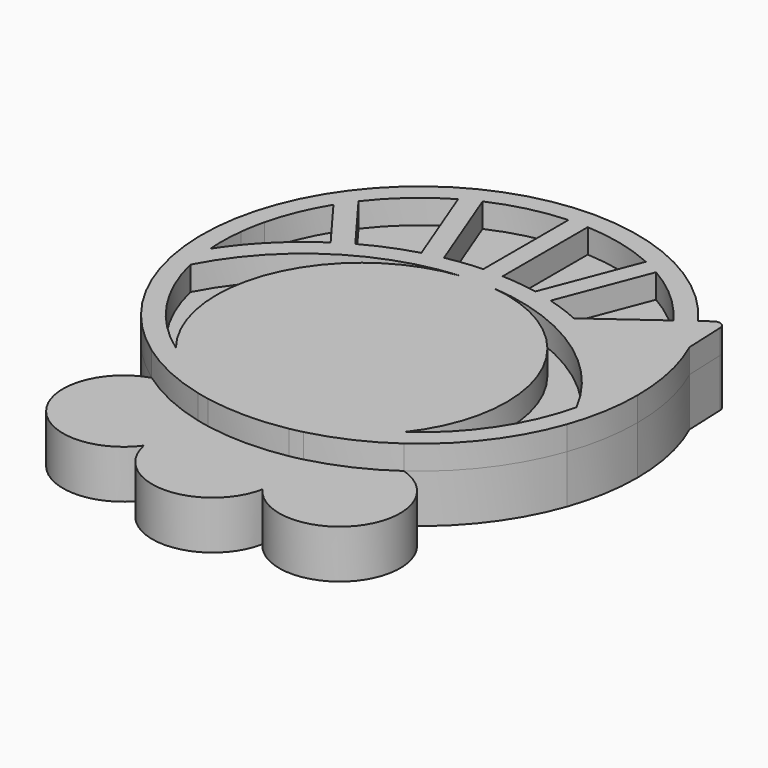
from build123d import *

# Parameters (mm, degrees)
F1_DEPTH = 2
F2_DEPTH = 1


with BuildPart() as f1:
    # F0 (on Top) → F1 (new body)
    with BuildSketch(Plane.XY):
        with BuildLine():
            ThreePointArc((7.2814781438, 5.28961965), (-6.3961147037, 6.3316440753), (-5.2155835522, -7.3346907372))
            ThreePointArc((-5.2155835522, -7.3346907372), (-3.7605276418, -8.1767005482), (-2.1742632903, -8.7334173806))
            ThreePointArc((-2.1742632903, -8.7334173806), (-1.9247980499, -8.7917661745), (-1.6737730699, -8.8429906542))
            ThreePointArc((-1.6737730699, -8.8429906542), (0, -9), (1.6737730699, -8.8429906542))
            ThreePointArc((1.6737730699, -8.8429906542), (1.9247980499, -8.7917661745), (2.1742632903, -8.7334173806))
            ThreePointArc((2.1742632903, -8.7334173806), (3.7605276418, -8.1767005482), (5.2155835522, -7.3346907372))
            ThreePointArc((5.2155835522, -7.3346907372), (7.1851103596, -5.4197960404), (8.4852813742, -3))
            Line((8.4852813742, -3), (8.2074613141, 3.6929092566))
            ThreePointArc((8.2074613141, 3.6929092566), (7.785511056, 4.5150656249), (7.2814781438, 5.28961965))
        make_face()
        with BuildLine():
            ThreePointArc((4.0924321005, 7.1057722664), (5.4838115432, 6.0965409011), (6.6342356421, 4.8194312366))
            ThreePointArc((6.6342356421, 4.8194312366), (7.7987413172, 2.5336996403), (8.2, 0))
            ThreePointArc((8.2, 0), (8.1945029875, -0.3002012451), (8.1780193201, -0.6))
            ThreePointArc((8.1780193201, -0.6), (8.1056933876, -1.2400543156), (7.9833517385, -1.8724569471))
            ThreePointArc((7.9833517385, -1.8724569471), (6.7951614423, -4.5897473758), (4.718116385, -6.7066666667))
            ThreePointArc((4.718116385, -6.7066666667), (0, -8.2), (-4.718116385, -6.7066666667))
            ThreePointArc((-4.718116385, -6.7066666667), (-6.7951614423, -4.5897473758), (-7.9833517385, -1.8724569471))
            ThreePointArc((-7.9833517385, -1.8724569471), (-8.1056933876, -1.2400543156), (-8.1780193201, -0.6))
            ThreePointArc((-8.1780193201, -0.6), (-8.19816566, 0.1734353216), (-8.1453273459, 0.945326625))
            ThreePointArc((-8.1453273459, 0.945326625), (-8.071860174, 1.4439783003), (-7.9678953297, 1.9371742346))
            ThreePointArc((-7.9678953297, 1.9371742346), (-7.5714581737, 3.148495057), (-6.992101102, 4.2837509475))
            ThreePointArc((-6.992101102, 4.2837509475), (-6.7619721437, 4.6385054412), (-6.5138611979, 4.9809248433))
            ThreePointArc((-6.5138611979, 4.9809248433), (-5.408521843, 6.1634317936), (-4.0924321005, 7.1057722664))
            ThreePointArc((-4.0924321005, 7.1057722664), (-3.7389698581, 7.2979520689), (-3.3765066945, 7.4725633181))
            ThreePointArc((-3.3765066945, 7.4725633181), (-1.9220470789, 7.9715578795), (-0.4, 8.1902380918))
            ThreePointArc((-0.4, 8.1902380918), (0, 8.2), (0.4, 8.1902380918))
            ThreePointArc((0.4, 8.1902380918), (1.9220470789, 7.9715578795), (3.3765066945, 7.4725633181))
            ThreePointArc((3.3765066945, 7.4725633181), (3.7389698581, 7.2979520689), (4.0924321005, 7.1057722664))
        make_face(mode=Mode.SUBTRACT)
        with BuildLine():
            ThreePointArc((-4.718116385, -6.7066666667), (0, -8.2), (4.718116385, -6.7066666667))
            ThreePointArc((4.718116385, -6.7066666667), (5.5357708849, -0.6858606979), (0.6763903311, 2.9617527725))
            ThreePointArc((0.6763903311, 2.9617527725), (0, 2.9872418814), (-0.6763903311, 2.9617527725))
            ThreePointArc((-0.6763903311, 2.9617527725), (-5.5357708849, -0.6858606979), (-4.718116385, -6.7066666667))
        make_face()
        with BuildLine():
            ThreePointArc((-2.1742632903, -8.7334173806), (-3.7605276418, -8.1767005482), (-5.2155835522, -7.3346907372))
            ThreePointArc((-5.2155835522, -7.3346907372), (-6.5031269408, -11.1771583895), (-2.4507149007, -11.1939599938))
            ThreePointArc((-2.4507149007, -11.1939599938), (-2.4421572707, -10.165333875), (-2.020134629, -9.2272284357))
            ThreePointArc((-2.020134629, -9.2272284357), (-2.0843920362, -8.976325602), (-2.1742632903, -8.7334173806))
        make_face()
        with BuildLine():
            ThreePointArc((2.020134629, -9.2272284357), (2.4421572707, -10.165333875), (2.4507149007, -11.1939599938))
            ThreePointArc((2.4507149007, -11.1939599938), (6.5031269408, -11.1771583895), (5.2155835522, -7.3346907372))
            ThreePointArc((5.2155835522, -7.3346907372), (3.7605276418, -8.1767005482), (2.1742632903, -8.7334173806))
            ThreePointArc((2.1742632903, -8.7334173806), (2.0843920362, -8.976325602), (2.020134629, -9.2272284357))
        make_face()
        with BuildLine():
            ThreePointArc((-2.020134629, -9.2272284357), (-2.028692259, -10.2558545545), (-2.4507149007, -11.1939599938))
            ThreePointArc((-2.4507149007, -11.1939599938), (0, -13.2), (2.4507149007, -11.1939599938))
            ThreePointArc((2.4507149007, -11.1939599938), (2.028692259, -10.2558545545), (2.020134629, -9.2272284357))
            ThreePointArc((2.020134629, -9.2272284357), (1.8569190048, -9.0261267044), (1.6737730699, -8.8429906542))
            ThreePointArc((1.6737730699, -8.8429906542), (0, -9), (-1.6737730699, -8.8429906542))
            ThreePointArc((-1.6737730699, -8.8429906542), (-1.8569190048, -9.0261267044), (-2.020134629, -9.2272284357))
        make_face()
        with BuildLine():
            ThreePointArc((8.1780193201, -0.6), (6.3564187379, 1.4589503838), (4.0346237711, 2.9309468158))
            ThreePointArc((4.0346237711, 2.9309468158), (3.3625359736, 3.2050720707), (2.6720023112, 3.4287010584))
            ThreePointArc((2.6720023112, 3.4287010584), (2.2814259241, 3.5307447638), (1.8869783621, 3.6166164872))
            ThreePointArc((1.8869783621, 3.6166164872), (1.1468403301, 3.732664448), (0.4, 3.7918333319))
            ThreePointArc((0.4, 3.7918333319), (0, 3.8), (-0.4, 3.7918333319))
            ThreePointArc((-0.4, 3.7918333319), (-1.1468403301, 3.732664448), (-1.8869783621, 3.6166164872))
            ThreePointArc((-1.8869783621, 3.6166164872), (-2.2814259241, 3.5307447638), (-2.6720023112, 3.4287010584))
            ThreePointArc((-2.6720023112, 3.4287010584), (-3.7242179593, 3.0647780222), (-4.7283647591, 2.5838550026))
            ThreePointArc((-4.7283647591, 2.5838550026), (-5.0763601287, 2.382754192), (-5.4158169003, 2.1675533241))
            ThreePointArc((-5.4158169003, 2.1675533241), (-6.2373110314, 1.5588326544), (-6.9909121579, 0.8678342439))
            ThreePointArc((-6.9909121579, 0.8678342439), (-7.2666228528, 0.5754233563), (-7.530112508, 0.2719538915))
            ThreePointArc((-7.530112508, 0.2719538915), (-7.8661570846, -0.1550386896), (-8.1780193201, -0.6))
            ThreePointArc((-8.1780193201, -0.6), (-8.1056933876, -1.2400543156), (-7.9833517385, -1.8724569471))
            ThreePointArc((-7.9833517385, -1.8724569471), (-4.9588485641, 1.4953543981), (-0.6763903311, 2.9617527725))
            ThreePointArc((-0.6763903311, 2.9617527725), (0, 2.9872418814), (0.6763903311, 2.9617527725))
            ThreePointArc((0.6763903311, 2.9617527725), (4.9588485641, 1.4953543981), (7.9833517385, -1.8724569471))
            ThreePointArc((7.9833517385, -1.8724569471), (8.1056933876, -1.2400543156), (8.1780193201, -0.6))
        make_face()
        with BuildLine():
            ThreePointArc((4.718116385, -6.7066666667), (6.7951614423, -4.5897473758), (7.9833517385, -1.8724569471))
            ThreePointArc((7.9833517385, -1.8724569471), (4.9588485641, 1.4953543981), (0.6763903311, 2.9617527725))
            ThreePointArc((0.6763903311, 2.9617527725), (5.5357708849, -0.6858606979), (4.718116385, -6.7066666667))
        make_face()
        with BuildLine():
            ThreePointArc((-7.9833517385, -1.8724569471), (-6.7951614423, -4.5897473758), (-4.718116385, -6.7066666667))
            ThreePointArc((-4.718116385, -6.7066666667), (-5.5357708849, -0.6858606979), (-0.6763903311, 2.9617527725))
            ThreePointArc((-0.6763903311, 2.9617527725), (-4.9588485641, 1.4953543981), (-7.9833517385, -1.8724569471))
        make_face()
        with BuildLine():
            Line((1.8869783621, 3.6166164872), (3.3765066945, 7.4725633181))
            ThreePointArc((3.3765066945, 7.4725633181), (1.9220470789, 7.9715578795), (0.4, 8.1902380918))
            Line((0.4, 8.1902380918), (0.4, 3.7918333319))
            ThreePointArc((0.4, 3.7918333319), (1.1468403301, 3.732664448), (1.8869783621, 3.6166164872))
        make_face()
        with BuildLine():
            Line((-0.4, 3.7918333319), (-0.4, 8.1902380918))
            ThreePointArc((-0.4, 8.1902380918), (-1.9220470789, 7.9715578795), (-3.3765066945, 7.4725633181))
            Line((-3.3765066945, 7.4725633181), (-1.8869783621, 3.6166164872))
            ThreePointArc((-1.8869783621, 3.6166164872), (-1.1468403301, 3.732664448), (-0.4, 3.7918333319))
        make_face()
        with BuildLine():
            Line((-2.6720023112, 3.4287010584), (-4.0924321005, 7.1057722664))
            ThreePointArc((-4.0924321005, 7.1057722664), (-5.408521843, 6.1634317936), (-6.5138611979, 4.9809248433))
            Line((-6.5138611979, 4.9809248433), (-4.7283647591, 2.5838550026))
            ThreePointArc((-4.7283647591, 2.5838550026), (-3.7242179593, 3.0647780222), (-2.6720023112, 3.4287010584))
        make_face()
        with BuildLine():
            ThreePointArc((8.2, 0), (7.7987413172, 2.5336996403), (6.6342356421, 4.8194312366))
            Line((6.6342356421, 4.8194312366), (4.0346237711, 2.9309468158))
            ThreePointArc((4.0346237711, 2.9309468158), (6.3564187379, 1.4589503838), (8.1780193201, -0.6))
            ThreePointArc((8.1780193201, -0.6), (8.1945029875, -0.3002012451), (8.2, 0))
        make_face()
        with BuildLine():
            Line((4.0346237711, 2.9309468158), (6.6342356421, 4.8194312366))
            ThreePointArc((6.6342356421, 4.8194312366), (5.4838115432, 6.0965409011), (4.0924321005, 7.1057722664))
            Line((4.0924321005, 7.1057722664), (2.6720023112, 3.4287010584))
            ThreePointArc((2.6720023112, 3.4287010584), (3.3625359736, 3.2050720707), (4.0346237711, 2.9309468158))
        make_face()
        with BuildLine():
            Line((-5.4158169003, 2.1675533241), (-6.992101102, 4.2837509475))
            ThreePointArc((-6.992101102, 4.2837509475), (-7.5714581737, 3.148495057), (-7.9678953297, 1.9371742346))
            Line((-7.9678953297, 1.9371742346), (-6.9909121579, 0.8678342439))
            ThreePointArc((-6.9909121579, 0.8678342439), (-6.2373110314, 1.5588326544), (-5.4158169003, 2.1675533241))
        make_face()
        with BuildLine():
            Line((0.4, 3.7918333319), (0.4, 8.1902380918))
            ThreePointArc((0.4, 8.1902380918), (0, 8.2), (-0.4, 8.1902380918))
            Line((-0.4, 8.1902380918), (-0.4, 3.7918333319))
            ThreePointArc((-0.4, 3.7918333319), (0, 3.8), (0.4, 3.7918333319))
        make_face()
        with BuildLine():
            Line((2.6720023112, 3.4287010584), (4.0924321005, 7.1057722664))
            ThreePointArc((4.0924321005, 7.1057722664), (3.7389698581, 7.2979520689), (3.3765066945, 7.4725633181))
            Line((3.3765066945, 7.4725633181), (1.8869783621, 3.6166164872))
            ThreePointArc((1.8869783621, 3.6166164872), (2.2814259241, 3.5307447638), (2.6720023112, 3.4287010584))
        make_face()
        with BuildLine():
            Line((-1.8869783621, 3.6166164872), (-3.3765066945, 7.4725633181))
            ThreePointArc((-3.3765066945, 7.4725633181), (-3.7389698581, 7.2979520689), (-4.0924321005, 7.1057722664))
            Line((-4.0924321005, 7.1057722664), (-2.6720023112, 3.4287010584))
            ThreePointArc((-2.6720023112, 3.4287010584), (-2.2814259241, 3.5307447638), (-1.8869783621, 3.6166164872))
        make_face()
        with BuildLine():
            ThreePointArc((9, 0), (8.7996349875, 1.8884978387), (8.2074613141, 3.6929092566))
            Line((8.2074613141, 3.6929092566), (8.4852813742, -3))
            ThreePointArc((8.4852813742, -3), (8.8703870369, -1.5219178085), (9, 0))
        make_face()
        with BuildLine():
            Line((-4.7283647591, 2.5838550026), (-6.5138611979, 4.9809248433))
            ThreePointArc((-6.5138611979, 4.9809248433), (-6.7619721437, 4.6385054412), (-6.992101102, 4.2837509475))
            Line((-6.992101102, 4.2837509475), (-5.4158169003, 2.1675533241))
            ThreePointArc((-5.4158169003, 2.1675533241), (-5.0763601287, 2.382754192), (-4.7283647591, 2.5838550026))
        make_face()
        with BuildLine():
            ThreePointArc((-7.9678953297, 1.9371742346), (-8.071860174, 1.4439783003), (-8.1453273459, 0.945326625))
            Line((-8.1453273459, 0.945326625), (-7.530112508, 0.2719538915))
            ThreePointArc((-7.530112508, 0.2719538915), (-7.2666228528, 0.5754233563), (-6.9909121579, 0.8678342439))
            Line((-6.9909121579, 0.8678342439), (-7.9678953297, 1.9371742346))
        make_face()
        with BuildLine():
            Line((7.6860047074, 5.5834874083), (7.2814781438, 5.28961965))
            ThreePointArc((7.2814781438, 5.28961965), (7.785511056, 4.5150656249), (8.2074613141, 3.6929092566))
            Line((8.2074613141, 3.6929092566), (8.1380607123, 5.3648257129))
            ThreePointArc((8.1380607123, 5.3648257129), (7.9774785182, 5.6094576733), (7.6860047074, 5.5834874083))
        make_face()
        with BuildLine():
            ThreePointArc((-2.020134629, -9.2272284357), (-2.4421572707, -10.165333875), (-2.4507149007, -11.1939599938))
            ThreePointArc((-2.4507149007, -11.1939599938), (-2.028692259, -10.2558545545), (-2.020134629, -9.2272284357))
        make_face()
        with BuildLine():
            ThreePointArc((2.020134629, -9.2272284357), (2.028692259, -10.2558545545), (2.4507149007, -11.1939599938))
            ThreePointArc((2.4507149007, -11.1939599938), (2.4421572707, -10.165333875), (2.020134629, -9.2272284357))
        make_face()
        with BuildLine():
            ThreePointArc((-8.1453273459, 0.945326625), (-8.19816566, 0.1734353216), (-8.1780193201, -0.6))
            ThreePointArc((-8.1780193201, -0.6), (-7.8661570846, -0.1550386896), (-7.530112508, 0.2719538915))
            Line((-7.530112508, 0.2719538915), (-8.1453273459, 0.945326625))
        make_face()
        with BuildLine():
            ThreePointArc((-1.6737730699, -8.8429906542), (-1.9247980499, -8.7917661745), (-2.1742632903, -8.7334173806))
            ThreePointArc((-2.1742632903, -8.7334173806), (-2.0843920362, -8.976325602), (-2.020134629, -9.2272284357))
            ThreePointArc((-2.020134629, -9.2272284357), (-1.8569190048, -9.0261267044), (-1.6737730699, -8.8429906542))
        make_face()
        with BuildLine():
            ThreePointArc((2.1742632903, -8.7334173806), (1.9247980499, -8.7917661745), (1.6737730699, -8.8429906542))
            ThreePointArc((1.6737730699, -8.8429906542), (1.8569190048, -9.0261267044), (2.020134629, -9.2272284357))
            ThreePointArc((2.020134629, -9.2272284357), (2.0843920362, -8.976325602), (2.1742632903, -8.7334173806))
        make_face()
    extrude(amount=F1_DEPTH)


with BuildPart() as f2:
    # F0 (on Top) → F2 (new body)
    with BuildSketch(Plane.XY):
        with BuildLine():
            ThreePointArc((7.2814781438, 5.28961965), (-6.3961147037, 6.3316440753), (-5.2155835522, -7.3346907372))
            ThreePointArc((-5.2155835522, -7.3346907372), (-3.7605276418, -8.1767005482), (-2.1742632903, -8.7334173806))
            ThreePointArc((-2.1742632903, -8.7334173806), (-1.9247980499, -8.7917661745), (-1.6737730699, -8.8429906542))
            ThreePointArc((-1.6737730699, -8.8429906542), (0, -9), (1.6737730699, -8.8429906542))
            ThreePointArc((1.6737730699, -8.8429906542), (1.9247980499, -8.7917661745), (2.1742632903, -8.7334173806))
            ThreePointArc((2.1742632903, -8.7334173806), (3.7605276418, -8.1767005482), (5.2155835522, -7.3346907372))
            ThreePointArc((5.2155835522, -7.3346907372), (7.1851103596, -5.4197960404), (8.4852813742, -3))
            Line((8.4852813742, -3), (8.2074613141, 3.6929092566))
            ThreePointArc((8.2074613141, 3.6929092566), (7.785511056, 4.5150656249), (7.2814781438, 5.28961965))
        make_face()
        with BuildLine():
            ThreePointArc((4.0924321005, 7.1057722664), (5.4838115432, 6.0965409011), (6.6342356421, 4.8194312366))
            ThreePointArc((6.6342356421, 4.8194312366), (7.7987413172, 2.5336996403), (8.2, 0))
            ThreePointArc((8.2, 0), (8.1945029875, -0.3002012451), (8.1780193201, -0.6))
            ThreePointArc((8.1780193201, -0.6), (8.1056933876, -1.2400543156), (7.9833517385, -1.8724569471))
            ThreePointArc((7.9833517385, -1.8724569471), (6.7951614423, -4.5897473758), (4.718116385, -6.7066666667))
            ThreePointArc((4.718116385, -6.7066666667), (0, -8.2), (-4.718116385, -6.7066666667))
            ThreePointArc((-4.718116385, -6.7066666667), (-6.7951614423, -4.5897473758), (-7.9833517385, -1.8724569471))
            ThreePointArc((-7.9833517385, -1.8724569471), (-8.1056933876, -1.2400543156), (-8.1780193201, -0.6))
            ThreePointArc((-8.1780193201, -0.6), (-8.19816566, 0.1734353216), (-8.1453273459, 0.945326625))
            ThreePointArc((-8.1453273459, 0.945326625), (-8.071860174, 1.4439783003), (-7.9678953297, 1.9371742346))
            ThreePointArc((-7.9678953297, 1.9371742346), (-7.5714581737, 3.148495057), (-6.992101102, 4.2837509475))
            ThreePointArc((-6.992101102, 4.2837509475), (-6.7619721437, 4.6385054412), (-6.5138611979, 4.9809248433))
            ThreePointArc((-6.5138611979, 4.9809248433), (-5.408521843, 6.1634317936), (-4.0924321005, 7.1057722664))
            ThreePointArc((-4.0924321005, 7.1057722664), (-3.7389698581, 7.2979520689), (-3.3765066945, 7.4725633181))
            ThreePointArc((-3.3765066945, 7.4725633181), (-1.9220470789, 7.9715578795), (-0.4, 8.1902380918))
            ThreePointArc((-0.4, 8.1902380918), (0, 8.2), (0.4, 8.1902380918))
            ThreePointArc((0.4, 8.1902380918), (1.9220470789, 7.9715578795), (3.3765066945, 7.4725633181))
            ThreePointArc((3.3765066945, 7.4725633181), (3.7389698581, 7.2979520689), (4.0924321005, 7.1057722664))
        make_face(mode=Mode.SUBTRACT)
        with BuildLine():
            ThreePointArc((-4.718116385, -6.7066666667), (0, -8.2), (4.718116385, -6.7066666667))
            ThreePointArc((4.718116385, -6.7066666667), (5.5357708849, -0.6858606979), (0.6763903311, 2.9617527725))
            ThreePointArc((0.6763903311, 2.9617527725), (0, 2.9872418814), (-0.6763903311, 2.9617527725))
            ThreePointArc((-0.6763903311, 2.9617527725), (-5.5357708849, -0.6858606979), (-4.718116385, -6.7066666667))
        make_face()
        with BuildLine():
            ThreePointArc((8.1780193201, -0.6), (6.3564187379, 1.4589503838), (4.0346237711, 2.9309468158))
            ThreePointArc((4.0346237711, 2.9309468158), (3.3625359736, 3.2050720707), (2.6720023112, 3.4287010584))
            ThreePointArc((2.6720023112, 3.4287010584), (2.2814259241, 3.5307447638), (1.8869783621, 3.6166164872))
            ThreePointArc((1.8869783621, 3.6166164872), (1.1468403301, 3.732664448), (0.4, 3.7918333319))
            ThreePointArc((0.4, 3.7918333319), (0, 3.8), (-0.4, 3.7918333319))
            ThreePointArc((-0.4, 3.7918333319), (-1.1468403301, 3.732664448), (-1.8869783621, 3.6166164872))
            ThreePointArc((-1.8869783621, 3.6166164872), (-2.2814259241, 3.5307447638), (-2.6720023112, 3.4287010584))
            ThreePointArc((-2.6720023112, 3.4287010584), (-3.7242179593, 3.0647780222), (-4.7283647591, 2.5838550026))
            ThreePointArc((-4.7283647591, 2.5838550026), (-5.0763601287, 2.382754192), (-5.4158169003, 2.1675533241))
            ThreePointArc((-5.4158169003, 2.1675533241), (-6.2373110314, 1.5588326544), (-6.9909121579, 0.8678342439))
            ThreePointArc((-6.9909121579, 0.8678342439), (-7.2666228528, 0.5754233563), (-7.530112508, 0.2719538915))
            ThreePointArc((-7.530112508, 0.2719538915), (-7.8661570846, -0.1550386896), (-8.1780193201, -0.6))
            ThreePointArc((-8.1780193201, -0.6), (-8.1056933876, -1.2400543156), (-7.9833517385, -1.8724569471))
            ThreePointArc((-7.9833517385, -1.8724569471), (-4.9588485641, 1.4953543981), (-0.6763903311, 2.9617527725))
            ThreePointArc((-0.6763903311, 2.9617527725), (0, 2.9872418814), (0.6763903311, 2.9617527725))
            ThreePointArc((0.6763903311, 2.9617527725), (4.9588485641, 1.4953543981), (7.9833517385, -1.8724569471))
            ThreePointArc((7.9833517385, -1.8724569471), (8.1056933876, -1.2400543156), (8.1780193201, -0.6))
        make_face()
        with BuildLine():
            ThreePointArc((8.2, 0), (7.7987413172, 2.5336996403), (6.6342356421, 4.8194312366))
            Line((6.6342356421, 4.8194312366), (4.0346237711, 2.9309468158))
            ThreePointArc((4.0346237711, 2.9309468158), (6.3564187379, 1.4589503838), (8.1780193201, -0.6))
            ThreePointArc((8.1780193201, -0.6), (8.1945029875, -0.3002012451), (8.2, 0))
        make_face()
        with BuildLine():
            Line((0.4, 3.7918333319), (0.4, 8.1902380918))
            ThreePointArc((0.4, 8.1902380918), (0, 8.2), (-0.4, 8.1902380918))
            Line((-0.4, 8.1902380918), (-0.4, 3.7918333319))
            ThreePointArc((-0.4, 3.7918333319), (0, 3.8), (0.4, 3.7918333319))
        make_face()
        with BuildLine():
            Line((-1.8869783621, 3.6166164872), (-3.3765066945, 7.4725633181))
            ThreePointArc((-3.3765066945, 7.4725633181), (-3.7389698581, 7.2979520689), (-4.0924321005, 7.1057722664))
            Line((-4.0924321005, 7.1057722664), (-2.6720023112, 3.4287010584))
            ThreePointArc((-2.6720023112, 3.4287010584), (-2.2814259241, 3.5307447638), (-1.8869783621, 3.6166164872))
        make_face()
        with BuildLine():
            Line((2.6720023112, 3.4287010584), (4.0924321005, 7.1057722664))
            ThreePointArc((4.0924321005, 7.1057722664), (3.7389698581, 7.2979520689), (3.3765066945, 7.4725633181))
            Line((3.3765066945, 7.4725633181), (1.8869783621, 3.6166164872))
            ThreePointArc((1.8869783621, 3.6166164872), (2.2814259241, 3.5307447638), (2.6720023112, 3.4287010584))
        make_face()
        with BuildLine():
            ThreePointArc((9, 0), (8.7996349875, 1.8884978387), (8.2074613141, 3.6929092566))
            Line((8.2074613141, 3.6929092566), (8.4852813742, -3))
            ThreePointArc((8.4852813742, -3), (8.8703870369, -1.5219178085), (9, 0))
        make_face()
        with BuildLine():
            Line((-4.7283647591, 2.5838550026), (-6.5138611979, 4.9809248433))
            ThreePointArc((-6.5138611979, 4.9809248433), (-6.7619721437, 4.6385054412), (-6.992101102, 4.2837509475))
            Line((-6.992101102, 4.2837509475), (-5.4158169003, 2.1675533241))
            ThreePointArc((-5.4158169003, 2.1675533241), (-5.0763601287, 2.382754192), (-4.7283647591, 2.5838550026))
        make_face()
        with BuildLine():
            Line((7.6860047074, 5.5834874083), (7.2814781438, 5.28961965))
            ThreePointArc((7.2814781438, 5.28961965), (7.785511056, 4.5150656249), (8.2074613141, 3.6929092566))
            Line((8.2074613141, 3.6929092566), (8.1380607123, 5.3648257129))
            ThreePointArc((8.1380607123, 5.3648257129), (7.9774785182, 5.6094576733), (7.6860047074, 5.5834874083))
        make_face()
    extrude(amount=F2_DEPTH)


with BuildPart() as f2_1:
    # F3: moved
    add(f2.part.moved(Location((0, 0, 2))))


solid = Compound([f1.part, f2_1.part])
